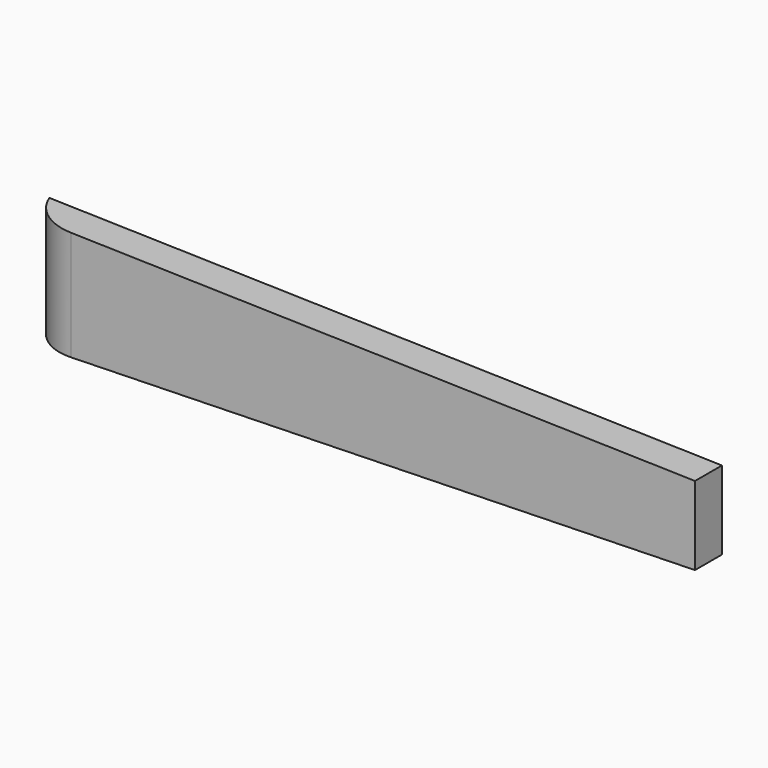
from build123d import *

# Parameters (mm, degrees)
F1_DEPTH    = 7.62
F2_T1_DEPTH = 80.1722009782
F3_R        = 2.54
F4_DEPTH    = 5.08


# Not quite as in the source:
# - a fillet or chamfer that OpenCascade refuses, or shapes differently, is made with other operations: its cross-section is extruded or revolved along the edge and cut away or added


with BuildPart() as f1:
    # F0 (on Front) → F1 (new body)
    with BuildSketch(Plane.XZ):
        Polygon((-48.8362722099, 5.4695218146), (-48.8362722099, -19.9304781854), (103.5160953464, -16.1204781854), (103.5160953464, 1.6595218146), align=None)
    extrude(amount=F1_DEPTH)

    # F2: fillet of radius 11.684 on 1 edges, made by hand

    # F2_s2 → F2_t1 (cut)
    with BuildSketch(Plane.XY.offset(-47.3165786745)):
        with BuildLine():
            ThreePointArc((-48.8362722099, 0), (-44.5538661868, -5.527653455), (-37.8818320142, -7.62))
            Line((-37.8818320142, -7.62), (-48.8362722099, -7.62))
            Line((-48.8362722099, -7.62), (-48.8362722099, 0))
        make_face()
    extrude(amount=F2_T1_DEPTH, mode=Mode.SUBTRACT)

    # F3 (on face) → F4 (cut)
    with BuildSketch(Plane(origin=(0, 0, 0), x_dir=(-1, 0, 0), z_dir=(0, 1, 0))):
        with Locations((40.8820770681, -7.3196464218)):
            Circle(F3_R)
    extrude(amount=-F4_DEPTH, mode=Mode.SUBTRACT)


solid = f1.part
